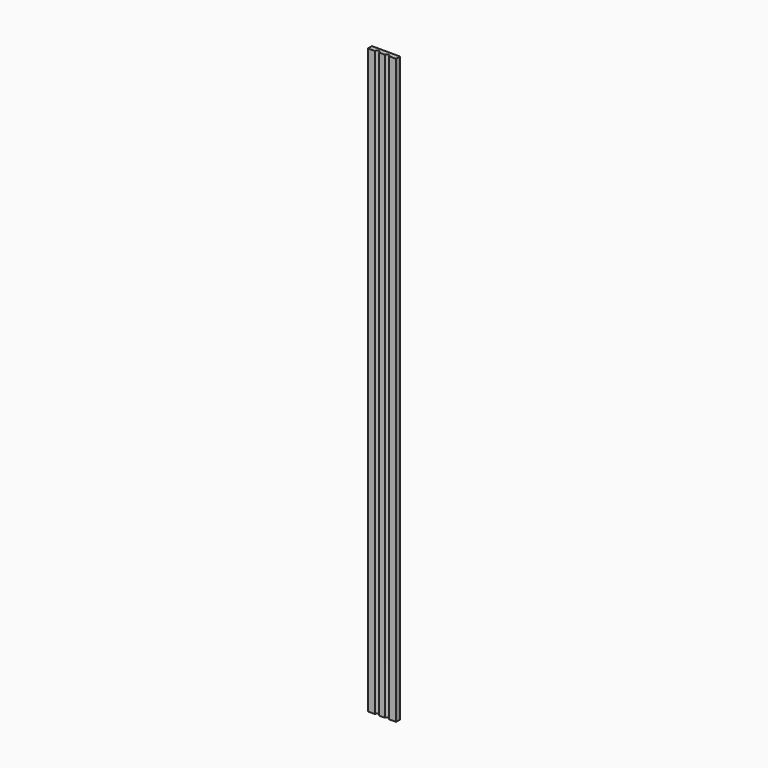
from build123d import *

# Parameters (mm, degrees)
F0_W     = 88.9
F0_H     = 1841.5
F1_DEPTH = 15.875
F3_DEPTH = 1841.5


# Not quite as in the source:
# - a length typed as a fraction of an inch, garbled in the dataset ("3 / 203.2 mm" for 3/8 in), is restored


with BuildPart() as f1:
    # F0 (on Front) → F1 (new body)
    with BuildSketch(Plane.XZ):
        with Locations((44.45, 920.75)):
            Rectangle(F0_W, F0_H)
    extrude(amount=F1_DEPTH)

    # F2 (on Top) → F3 (cut)
    with BuildSketch(Plane.XY):
        with BuildLine():
            Line((22.225, -15.875), (34.925, -15.875))
            ThreePointArc((34.925, -15.875), (28.575, -9.525), (22.225, -15.875))
        make_face()
        with BuildLine():
            Line((53.975, -15.875), (66.675, -15.875))
            ThreePointArc((66.675, -15.875), (60.325, -9.525), (53.975, -15.875))
        make_face()
    extrude(amount=F3_DEPTH, mode=Mode.SUBTRACT)


solid = f1.part
